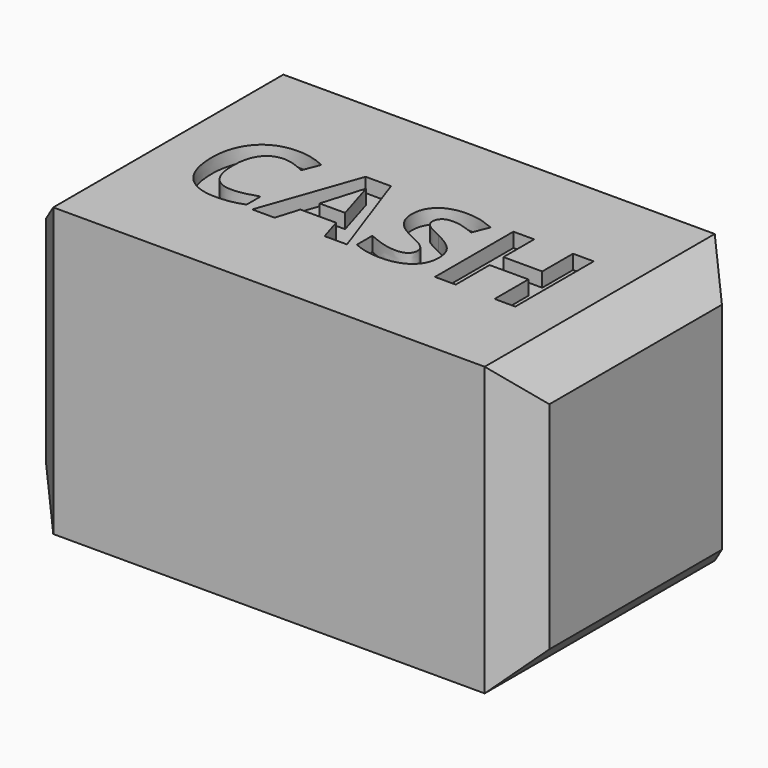
from build123d import *

# Parameters (mm, degrees)
F0_W         = 88.9
F0_H         = 50.8
F1_DEPTH     = 25.4
F2_SIZE      = 6.35
F4_DEPTH     = 6.35
F5_TEXT_SIZE = 24.2583417895
F6_DEPTH     = 2.54


# Not quite as in the source:
# - Text() gives the source's letters only with a copy of the font that has no kerning and outlines rounded to 1/6400 em; it was checked with that copy


with BuildPart() as f1:
    # F0 (on Front) → F1 (new body, symmetric)
    with BuildSketch(Plane.XZ):
        with Locations((0, 25.4)):
            Rectangle(F0_W, F0_H)
    extrude(amount=F1_DEPTH, both=True)

    # F2
    f2_edges = [f1.edges().sort_by_distance(p)[0] for p in [
        (-44.45, -25.4, 25.4),
        (-44.45, 0, 50.8),
        (-44.45, 25.4, 25.4),
        (-44.45, 0, 0),
        (44.45, 25.4, 25.4),
        (44.45, 0, 50.8),
        (44.45, -25.4, 25.4),
        (44.45, 0, 0),
    ]]
    chamfer(f2_edges, length=F2_SIZE)

    # F3 (on face) → F4 (cut)
    with BuildSketch(Plane(origin=(0, 0, 0), x_dir=(1, 0, 0), z_dir=(0, 0, -1))):
        with BuildLine():
            Line((12.7, 6.35), (-12.7, 6.35))
            ThreePointArc((-12.7, 6.35), (-19.05, 0), (-12.7, -6.35))
            Line((-12.7, -6.35), (12.7, -6.35))
            ThreePointArc((12.7, -6.35), (19.05, 0), (12.7, 6.35))
        make_face()
    extrude(amount=-F4_DEPTH, mode=Mode.SUBTRACT)

    # F5 (on face) → F6 (cut)
    with BuildSketch(Plane.XY.offset(50.8)):
        with Locations((-31.75, -8.7330030442)):
            Text('CASH', F5_TEXT_SIZE, font='Open Sans', font_style=FontStyle.BOLD, text_align=(TextAlign.LEFT, TextAlign.BOTTOM))
    extrude(amount=-F6_DEPTH, mode=Mode.SUBTRACT)


solid = f1.part
